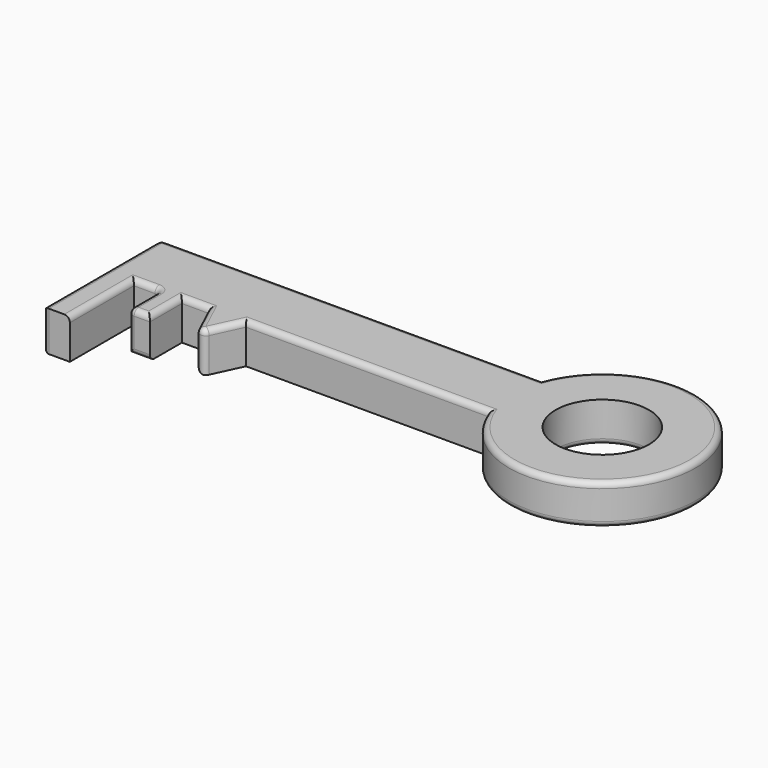
from build123d import *

# Parameters (mm, degrees)
F0_R     = 17.5
F0_W     = 10
F0_H     = 30
F0_W_2   = 8
F0_H_2   = 15
F1_DEPTH = 15
F2_R     = 2.1


with BuildPart() as f1:
    # F0 (on Top) → F1 (new body)
    with BuildSketch(Plane.XY):
        Polygon((29.2293787445, 29.4917059159), (-113.5933991075, 29.4917059159), (-113.5933991075, 4.4917059159), (-103.5933991075, 4.4917059159), (-93.5933991075, 4.4917059159), (-85.5933991075, 4.4917059159), (-75.5933991075, 4.4917059159), (-61.5933991075, 4.4917059159), (29.2293787445, 4.4917059159), align=None)
        with BuildLine():
            ThreePointArc((29.2293787445, 4.4917059159), (96.9211208211, 16.9917059159), (29.2293787445, 29.4917059159))
            Line((29.2293787445, 29.4917059159), (29.2293787445, 4.4917059159))
        make_face()
        with Locations((61.9211208211, 16.9917059159)):
            Circle(F0_R, mode=Mode.SUBTRACT)
        with Locations((-108.5933991075, -10.5082940841)):
            Rectangle(F0_W, F0_H)
        Polygon((-68.5933991075, -10.5082940841), (-61.5933991075, 4.4917059159), (-75.5933991075, 4.4917059159), align=None)
        with Locations((-89.5933991075, -3.0082940841)):
            Rectangle(F0_W_2, F0_H_2)
    extrude(amount=F1_DEPTH)

    # F2
    f2_edges = [f1.edges().sort_by_distance(p)[0] for p in [
        (-113.593399, 1.991706, 0),
        (-113.593399, 29.491706, 7.5),
        (-113.593399, 1.991706, 15),
        (-113.593399, -25.508294, 7.5),
        (-42.18201, 29.491706, 0),
        (-16.18201, 4.491706, 15),
        (-42.18201, 29.491706, 15),
        (96.921121, 16.991706, 15),
        (96.921121, 16.991706, 0),
        (-65.093399, -3.008294, 15),
        (-85.593399, -3.008294, 15),
        (-80.593399, 4.491706, 15),
        (-72.093399, -3.008294, 15),
        (-89.593399, -10.508294, 15),
        (-93.593399, 4.491706, 7.5),
        (-103.593399, -10.508294, 15),
        (-93.593399, -10.508294, 7.5),
        (-89.593399, -10.508294, 0),
        (-72.093399, -3.008294, 0),
        (-68.593399, -10.508294, 7.5),
        (-98.593399, 4.491706, 15),
        (44.421121, 16.991706, 0),
        (-93.593399, -3.008294, 15),
    ]]
    fillet(f2_edges, radius=F2_R)


solid = f1.part
